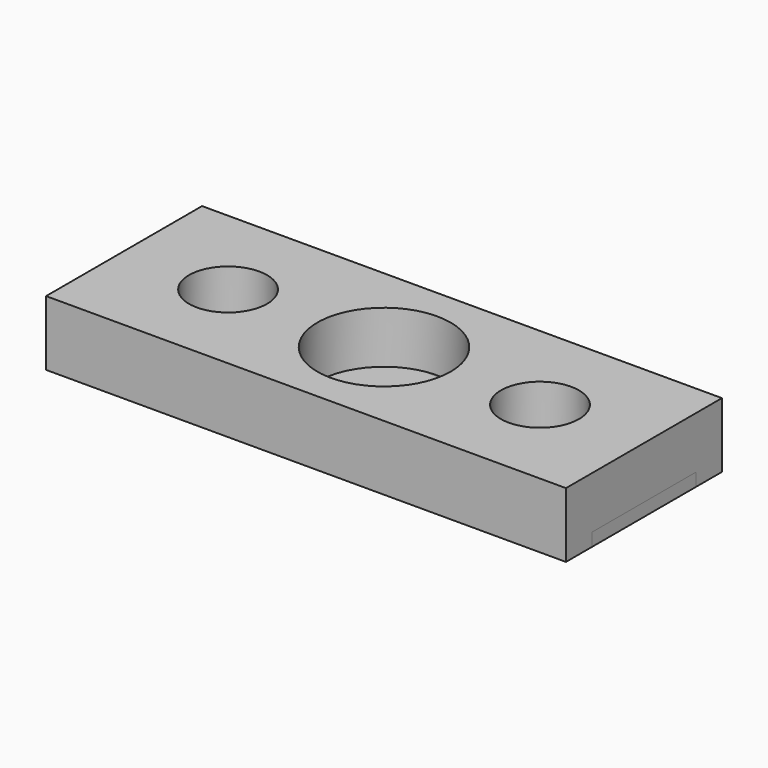
from build123d import *

# Parameters (mm, degrees)
F0_W     = 40
F0_H     = 15
F0_R     = 3
F0_R_2   = 5.125
F1_DEPTH = 1
F2_DEPTH = 5
F3_W     = 40
F3_H     = 10
F3_R     = 1.65
F4_DEPTH = 1
F5_DEPTH = 4


with BuildPart() as f1:
    # F0 (on Top) → F1 (new body)
    with BuildSketch(Plane.XY):
        Rectangle(F0_W, F0_H)
        with Locations((-12, 0)):
            Circle(F0_R, mode=Mode.SUBTRACT)
        Circle(F0_R_2, mode=Mode.SUBTRACT)
        with Locations((12, 0)):
            Circle(F0_R, mode=Mode.SUBTRACT)
        Circle(F0_R_2)
        Circle(F0_R, mode=Mode.SUBTRACT)
    extrude(amount=F1_DEPTH)

    # F0 (on Top) → F2 (join)
    with BuildSketch(Plane.XY):
        Rectangle(F0_W, F0_H)
        with Locations((-12, 0)):
            Circle(F0_R, mode=Mode.SUBTRACT)
        Circle(F0_R_2, mode=Mode.SUBTRACT)
        with Locations((12, 0)):
            Circle(F0_R, mode=Mode.SUBTRACT)
    extrude(amount=F2_DEPTH)


with BuildPart() as f4:
    # F3 (on Top) → F4 (new body)
    with BuildSketch(Plane.XY):
        Rectangle(F3_W, F3_H)
        with Locations((-8, 0)):
            Circle(F3_R, mode=Mode.SUBTRACT)
        with Locations((-8, 0)):
            Circle(F3_R)
    extrude(amount=F4_DEPTH)

    # F3 (on Top) → F5 (join)
    with BuildSketch(Plane.XY):
        with Locations((-8, 0)):
            Circle(F3_R)
    extrude(amount=F5_DEPTH)


solid = Compound([f1.part, f4.part])
